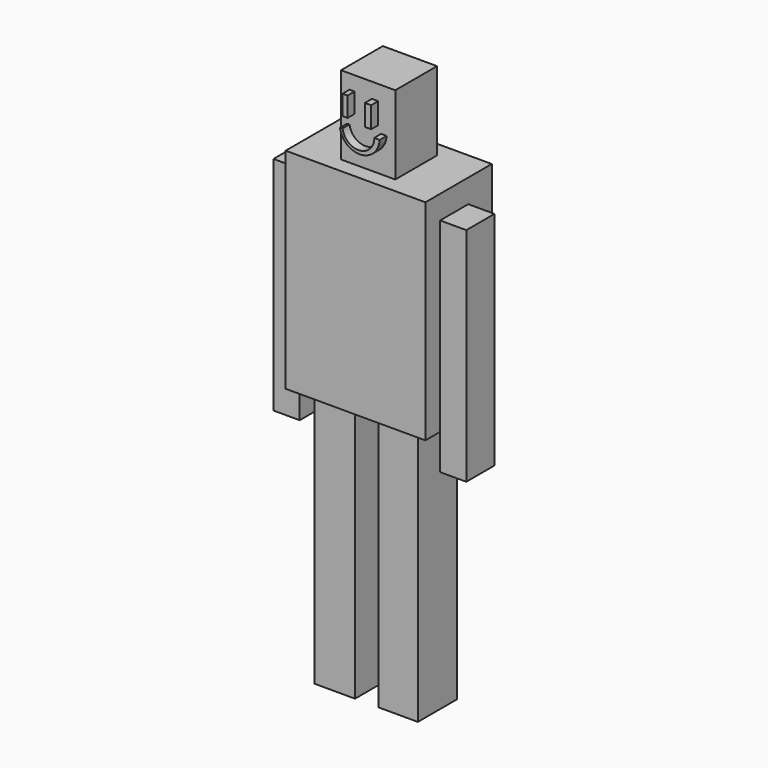
from build123d import *

# Parameters (mm, degrees)
F0_W     = 406.4
F0_H     = 609.6
F1_DEPTH = 241.3
F2_W     = 157.7554345131
F2_H     = 151.9362496853
F3_DEPTH = 228.6
F4_W     = 102.4757102132
F4_H     = 542.9573820229
F4_H_2   = 101.385278881
F5_DEPTH = 76.2
F6_W     = 117.2105111182
F6_H     = 141.6197903454
F6_W_2   = 115.0653380901
F6_H_2   = 142.1200931072
F7_DEPTH = 762
F8_W     = 14.6603360772
F8_H     = 57.432115078
F8_W_2   = 18.2616543025
F8_H_2   = 61.538875103
F9_DEPTH = 25.4


# Not quite as in the source:
# - a pattern or mirror of a feature is missing from the dataset's text; its kind, count and spacing are read off the source's solid


with BuildPart() as f1:
    # F0 (on Front) → F1 (new body)
    with BuildSketch(Plane.XZ):
        with Locations((-0.9644478559, 82.7934837226)):
            Rectangle(F0_W, F0_H)
    extrude(amount=F1_DEPTH)

    # F2 (on face) → F3 (join)
    with BuildSketch(Plane.XY.offset(387.5934837226)):
        with Locations((0, -120.65)):
            Rectangle(F2_W, F2_H)
    extrude(amount=F3_DEPTH)

    # F4 (on face) → F5 (join)
    with BuildSketch(Plane(origin=(-204.1644478559, 0, 0), x_dir=(0, -1, 0), z_dir=(-1, 0, 0))):
        with Locations((138.9757506549, 49.4721747341)):
            Rectangle(F4_W, F4_H)
        with Locations((138.9757506549, -272.6991557179)):
            Rectangle(F4_W, F4_H_2)
    f5 = extrude(amount=F5_DEPTH)

    # F5_copies: F5 across plane
    add(f5.mirror(Plane(origin=(0, 0, 0), x_dir=(0, 0, 1), z_dir=(1, 0, 0))))

    # F6 (on face) → F7 (join)
    with BuildSketch(Plane(origin=(0, 0, -222.0065162774), x_dir=(1, 0, 0), z_dir=(0, 0, -1))):
        with Locations((-101.9190382212, 119.4037105888)):
            Rectangle(F6_W, F6_H)
        with Locations((81.9740435109, 119.1535592079)):
            Rectangle(F6_W_2, F6_H_2)
    extrude(amount=F7_DEPTH)

    # F8 (on face) → F9 (join)
    with BuildSketch(Plane.XZ.offset(196.6181248426)):
        with Locations((-46.77233845, 545.7714498043)):
            Rectangle(F8_W, F8_H)
        with Locations((20.0242409483, 541.19977355)):
            Rectangle(F8_W_2, F8_H_2)
        with BuildLine():
            Line((-54.1025064886, 485.6823980808), (-61.6828501225, 484.8566651344))
            ThreePointArc((-61.6828501225, 484.8566651344), (-1.2605522205, 435.5338821249), (53.6077916622, 490.9690320492))
            Line((53.6077916622, 490.9690320492), (38.3146069944, 491.5615320206))
            ThreePointArc((38.3146069944, 491.5615320206), (-5.1247496202, 445.0914918544), (-54.1025064886, 485.6823980808))
        make_face()
    extrude(amount=F9_DEPTH)


solid = f1.part
